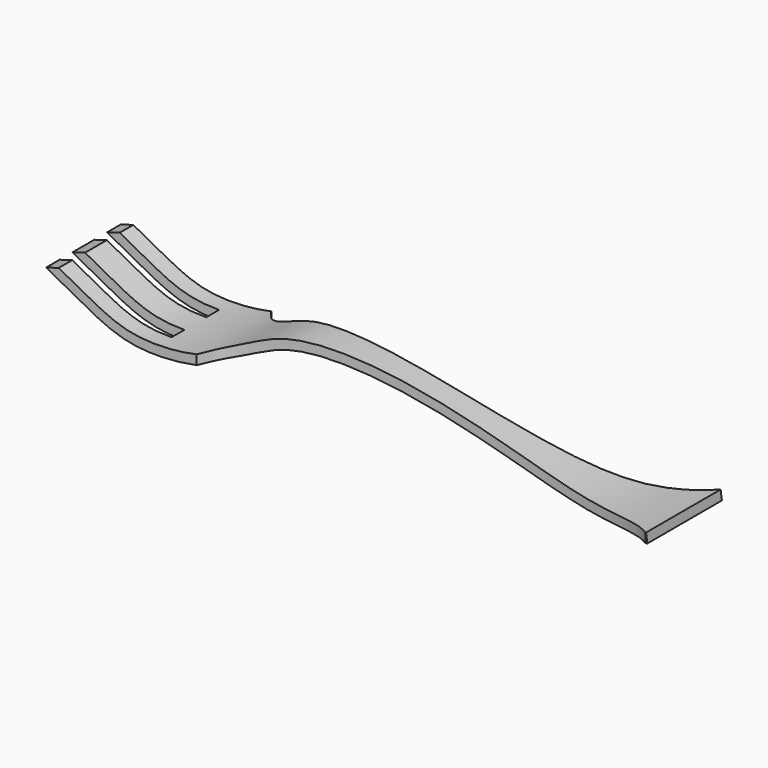
from build123d import *

# Parameters (mm, degrees)
F1_DEPTH      = 25.4
F3_DEPTH      = 25.4
F4_W          = 39.0272449004
F4_H          = 4.3723583221
F5_DEPTH      = 25.4
F5_DEPTH_BACK = 25.4
F6_T1_DEPTH   = 33.5402773225
F6_T3_DEPTH   = 30.7376088762
F6_T5_DEPTH   = 30.7376088762


# Not quite as in the source:
# - a fillet or chamfer that OpenCascade refuses, or shapes differently, is made with other operations: its cross-section is extruded or revolved along the edge and cut away or added
# - the dataset's text gives a spline's control points without its knots; the knots are read off the source's solid


with BuildPart() as f1:
    # F0 (on Front) → F1 (new body)
    with BuildSketch(Plane.XZ):
        with BuildLine():
            add(Edge.make_bspline(
                [(0, 0), (4.4898795982, -2.430600393), (13.2318122513, -7.1630535641), (25.2079192478, -13.3244586408), (46.747809493, -11.1510841184), (59.8226169022, -2.2642683961), (89.7594633376, -4.0178282037), (123.9327479047, -12.496915753), (146.5184579427, -16.4227730632), (158.7788514037, -14.6681828652), (164.518315, -13.8468057537)],
                knots=[0, 0, 0, 0, 0.1064534698, 0.2072681556, 0.3310783578, 0.4391158778, 0.5868054033, 0.7533079232, 0.8845159253, 1, 1, 1, 1], degree=3))
            Line((0, 0), (-1.2092138467, -2.2336969071))
            add(Edge.make_bspline(
                [(-1.2092138467, -2.2336969071), (0.1088149386, -2.9472129856), (2.7460517583, -4.3748817005), (6.0040545149, -6.1318835046), (8.5628225115, -7.5035818498), (10.1367651015, -8.3430408933), (11.3785170568, -9.0020171029), (12.6048560586, -9.650920119), (14.138765381, -10.4540097116), (16.02030758, -11.382465517), (17.97764057, -12.2500668756), (20.0431073063, -13.0280483508), (22.244592964, -13.6857569942), (24.6063765164, -14.1952550109), (27.1499357811, -14.5259664023), (29.8089625219, -14.6798707712), (33.4676391926, -14.6713272759), (37.2139158819, -14.3606756814), (40.8826729802, -13.7784351906), (43.55337076, -13.2110441914), (45.6783515747, -12.6330632536), (47.297100451, -12.1070220661), (48.8398454258, -11.551126362), (50.64857827, -10.8156324674), (52.67330894, -9.9182065503), (54.6063555942, -9.0502569259), (56.5050506802, -8.2482783972), (58.1105468575, -7.6588307529), (59.4440615397, -7.2464777671), (60.4768934024, -6.9699222274), (61.5571063422, -6.7286211329), (63.0810120698, -6.4498995564), (65.1245667249, -6.1840889422), (67.7763378106, -5.9942396899), (71.5443776217, -5.9064775805), (76.6313407164, -6.0902889762), (83.1624023854, -6.716231492), (89.9481280232, -7.676846362), (99.1417366838, -9.3048693233), (108.3525709149, -11.280700091), (117.1650295561, -13.2583818293), (123.4789786056, -14.656337098), (129.3922312538, -15.8803590881), (134.9726375944, -16.8775117712), (140.3050762278, -17.595644562), (144.6033320485, -17.9160432377), (147.9960763231, -17.974065639), (151.3366602177, -17.899910767), (155.4199316022, -17.6020128408), (160.1992114188, -17.0308928495), (163.3250500455, -16.5834529422), (164.8781493608, -16.3611882291)],
                knots=[0, 0, 0, 0, 0.03125, 0.0625, 0.078125, 0.09375, 0.1015625, 0.109375, 0.125, 0.140625, 0.15625, 0.171875, 0.1875, 0.203125, 0.21875, 0.234375, 0.25, 0.28125, 0.296875, 0.3125, 0.328125, 0.3359375, 0.34375, 0.359375, 0.375, 0.390625, 0.40625, 0.421875, 0.4296875, 0.4375, 0.4453125, 0.453125, 0.46875, 0.484375, 0.5, 0.53125, 0.5625, 0.59375, 0.625, 0.6875, 0.71875, 0.75, 0.78125, 0.8125, 0.84375, 0.875, 0.890625, 0.90625, 0.9375, 0.96875, 1, 1, 1, 1], degree=3))
            Line((164.8781493608, -16.3611882291), (164.518315, -13.8468057537))
        make_face()
    extrude(amount=F1_DEPTH)

    # F2 (on Top) → F3 (cut)
    with BuildSketch(Plane.XY):
        with BuildLine():
            add(Edge.make_bspline(
                [(42.06633138, -25.4), (43.0735812016, -24.0471734252), (45.7042675809, -19.7168059838), (59.0739423106, -17.3725118353), (101.1430071979, -15.1843665681), (137.8792590303, -17.5264103006), (159.6447736634, -21.7132412052), (164.3137633801, -25.4)],
                knots=[0, 0, 0, 0, 0.1009194512, 0.2480539867, 0.5214170371, 0.7890126938, 1, 1, 1, 1], degree=3))
            Line((42.06633138, -25.4), (164.3137633801, -25.4))
        make_face()
        with BuildLine():
            Line((164.3137633801, 0), (42.06633138, 0))
            add(Edge.make_bspline(
                [(42.06633138, 0), (43.0735812016, -1.3528265748), (45.7042675809, -5.6831940162), (59.0739423106, -8.0274881647), (101.1430071979, -10.2156334319), (137.8792590303, -7.8735896994), (159.6447736634, -3.6867587948), (164.3137633801, 0)],
                knots=[0, 0, 0, 0, 0.1009194512, 0.2480539867, 0.5214170371, 0.7890126938, 1, 1, 1, 1], degree=3))
        make_face()
    extrude(amount=-F3_DEPTH, mode=Mode.SUBTRACT)

    # F4 (on Top) → F5 (cut, two sides)
    with BuildSketch(Plane.XY) as f5_sk:
        with Locations((12.0170111186, -6.8037174642)):
            Rectangle(F4_W, F4_H)
        with Locations((12.0170111186, -18.5962825358)):
            Rectangle(F4_W, F4_H)
    extrude(amount=-F5_DEPTH, mode=Mode.SUBTRACT)
    extrude(f5_sk.sketch, amount=F5_DEPTH_BACK, mode=Mode.SUBTRACT)

    # F6: chamfer of 5.08 on 3 edges, made by hand

    # F6_s2 → F6_t1 (cut)
    with BuildSketch(Plane.XZ.offset(-4.0701386613)):
        with BuildLine():
            Line((4.6583858969, -2.3564008136), (-2.6123408892, -4.5239361786))
            Line((-2.6123408892, -4.5239361786), (-2.7016887655, -4.4755676248))
            ThreePointArc((-2.7016887655, -4.4755676248), (-1.3323720501, -2.2477838264), (-0.0893478763, 0.0483685539))
            Line((-0.0893478763, 0.0483685539), (0.0483685539, 0.0893478763))
            ThreePointArc((0.0483685539, 0.0893478763), (2.3430375646, -1.1526099074), (4.7066633214, -2.2670036645))
            Line((4.7066633214, -2.2670036645), (4.6583858969, -2.3564008136))
        make_face()
    extrude(amount=F6_T1_DEPTH, mode=Mode.SUBTRACT)

    # F6_s4 → F6_t3 (cut)
    with BuildSketch(Plane.XZ.offset(-13.0600352865)):
        with BuildLine():
            Line((4.6583858969, -2.3564008136), (-2.6123408892, -4.5239361786))
            Line((-2.6123408892, -4.5239361786), (-2.7016887655, -4.4755676248))
            ThreePointArc((-2.7016887655, -4.4755676248), (-1.3323720501, -2.2477838264), (-0.0893478763, 0.0483685539))
            Line((-0.0893478763, 0.0483685539), (0.0483685539, 0.0893478763))
            ThreePointArc((0.0483685539, 0.0893478763), (2.3430375646, -1.1526099074), (4.7066633214, -2.2670036645))
            Line((4.7066633214, -2.2670036645), (4.6583858969, -2.3564008136))
        make_face()
    extrude(amount=F6_T3_DEPTH, mode=Mode.SUBTRACT)

    # F6_s6 → F6_t5 (cut)
    with BuildSketch(Plane.XZ.offset(7.7224264103)):
        with BuildLine():
            Line((4.6583858969, -2.3564008136), (-2.6123408892, -4.5239361786))
            Line((-2.6123408892, -4.5239361786), (-2.7016887655, -4.4755676248))
            ThreePointArc((-2.7016887655, -4.4755676248), (-1.3323720501, -2.2477838264), (-0.0893478763, 0.0483685539))
            Line((-0.0893478763, 0.0483685539), (0.0483685539, 0.0893478763))
            ThreePointArc((0.0483685539, 0.0893478763), (2.3430375646, -1.1526099074), (4.7066633214, -2.2670036645))
            Line((4.7066633214, -2.2670036645), (4.6583858969, -2.3564008136))
        make_face()
    extrude(amount=F6_T5_DEPTH, mode=Mode.SUBTRACT)


solid = f1.part
